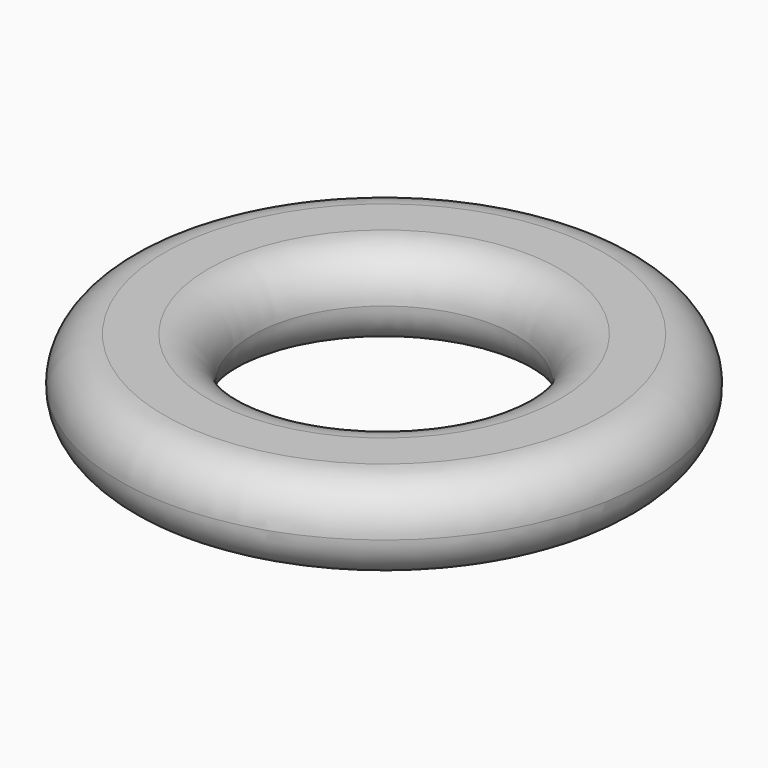
from build123d import *

# Parameters (mm, degrees)
F0_R     = 15
F0_R_2   = 7.5
F1_DEPTH = 5
F2_R     = 2.49999


# Not quite as in the source:
# - a fillet or chamfer is up to 0.001 mm smaller than in the source, because OpenCascade refuses the exact size


with BuildPart() as f1:
    # F0 (on Top) → F1 (new body)
    with BuildSketch(Plane.XY):
        Circle(F0_R)
        Circle(F0_R_2, mode=Mode.SUBTRACT)
    extrude(amount=F1_DEPTH)

    # F2 (radius 2.5 in the source; OpenCascade refuses exactly that, so slightly less here)
    f2_edges = [f1.edges().sort_by_distance(p)[0] for p in [
        (-15, 0, 5),
        (-15, 0, 0),
        (-7.5, 0, 5),
        (-7.5, 0, 0),
    ]]
    fillet(f2_edges, radius=F2_R)


solid = f1.part
